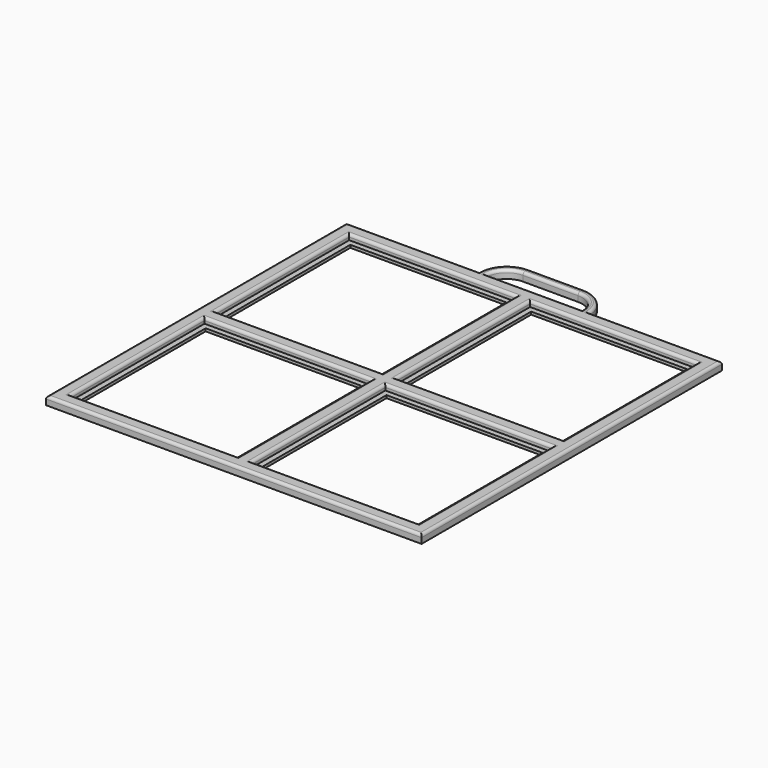
from build123d import *

# Parameters (mm, degrees)
F0_W         = 2.5711264648
F0_H         = 5
F1_DEPTH     = 3
F0_W_2       = 56.75
F0_H_2       = 56.75
F2_DEPTH     = 1
F3_R         = 1
F6_DEPTH     = 3
F7_T1_DEPTH  = 12.5
F7_T3_DEPTH  = 7.5711264648
F7_T5_DEPTH  = 3.5
F7_T8_ANGLE  = 90
F7_T10_ANGLE = 90


# Not quite as in the source:
# - a fillet or chamfer that OpenCascade refuses, or shapes differently, is made with other operations: its cross-section is extruded or revolved along the edge and cut away or added
# - a feature names something its author has since deleted; it is built from what else it names


with BuildPart() as f1:
    # F0 (on Top) → F1 (new body)
    with BuildSketch(Plane.XY):
        Polygon((-63.25, -34.2033516131), (-63.25, 26.5466483869), (-20, 26.5466483869), (-20, 31.5466483869), (-34.125, 31.5466483869), (-68.25, 31.5466483869), (-68.25, -36.7033516131), (0, -36.7033516131), (0, 31.5466483869), (-17.4288735352, 31.5466483869), (-17.4288735352, 26.5466483869), (-2.5, 26.5466483869), (-2.5, -34.2033516131), align=None)
        with Locations((-18.7144367676, 29.0466483869)):
            Rectangle(F0_W, F0_H)
    extrude(amount=F1_DEPTH)

    # F0 (on Top) → F2 (join)
    with BuildSketch(Plane.XY):
        Polygon((-20, 26.5466483869), (-63.25, 26.5466483869), (-63.25, -34.2033516131), (-2.5, -34.2033516131), (-2.5, 26.5466483869), (-17.4288735352, 26.5466483869), align=None)
        with Locations((-32.875, -3.8283516131)):
            Rectangle(F0_W_2, F0_H_2, mode=Mode.SUBTRACT)
    extrude(amount=F2_DEPTH)

    # F3
    f3_edges = [f1.edges().sort_by_distance(p)[0] for p in [
        (-32.875, 26.546648, 3),
        (-63.25, -3.828352, 3),
        (-32.875, -34.203352, 3),
        (-2.5, -3.828352, 3),
        (-34.125, 31.546648, 3),
        (-68.25, -2.578352, 3),
    ]]
    fillet(f3_edges, radius=F3_R)

    # F4: F1 across plane


with BuildPart() as f1_1:
    add(f1.part)
    add(f1.part.mirror(Plane.YZ))

    # F5: F1 across face


with BuildPart() as f1_2:
    add(f1_1.part)
    add(f1_1.part.mirror(Plane(origin=(0, -36.7033516131, 1.4986605371), x_dir=(1, 0, 0), z_dir=(0, -1, 0))))

    # F0 (on Top) → F6 (join)
    with BuildSketch(Plane.XY):
        with BuildLine():
            ThreePointArc((-10, 41.5466483869), (-17.0710678119, 38.6177161988), (-20, 31.5466483869))
            Line((-20, 31.5466483869), (-17.4288735352, 31.5466483869))
            ThreePointArc((-17.4288735352, 31.5466483869), (-15.2530068533, 36.7996552402), (-10, 38.9755219221))
            Line((-10, 38.9755219221), (0, 38.9755219221))
            Line((0, 38.9755219221), (0, 41.5466483869))
            Line((0, 41.5466483869), (-10, 41.5466483869))
        make_face()
        with Locations((-18.7144367676, 29.0466483869)):
            Rectangle(F0_W, F0_H)
    extrude(amount=F6_DEPTH)

    # F7: fillet of radius 1 on 4 edges, made by hand

    # F7_s2 → F7_t1 (cut)
    with BuildSketch(Plane.YZ.offset(-10)):
        with BuildLine():
            ThreePointArc((39.9755219221, 3), (39.2684151409, 2.7071067812), (38.9755219221, 2))
            Line((38.9755219221, 2), (38.9755219221, 3))
            Line((38.9755219221, 3), (39.9755219221, 3))
        make_face()
        with BuildLine():
            ThreePointArc((40.5466483869, 3), (41.2537551681, 2.7071067812), (41.5466483869, 2))
            Line((41.5466483869, 2), (41.5466483869, 3))
            Line((41.5466483869, 3), (40.5466483869, 3))
        make_face()
    extrude(amount=F7_T1_DEPTH, mode=Mode.SUBTRACT)

    # F7_s4 → F7_t3 (cut)
    with BuildSketch(Plane.YZ.offset(-22.5)):
        with BuildLine():
            ThreePointArc((27.5466483869, 3), (26.8395416057, 2.7071067812), (26.5466483869, 2))
            Line((26.5466483869, 2), (26.5466483869, 3))
            Line((26.5466483869, 3), (27.5466483869, 3))
        make_face()
    extrude(amount=F7_T3_DEPTH, mode=Mode.SUBTRACT)

    # F7_s6 → F7_t5 (cut)
    with BuildSketch(Plane.XZ.offset(-31.5466483869)):
        with BuildLine():
            ThreePointArc((-19, 3), (-19.7071067812, 2.7071067812), (-20, 2))
            Line((-20, 2), (-20, 3))
            Line((-20, 3), (-19, 3))
        make_face()
        with BuildLine():
            ThreePointArc((-18.4288735352, 3), (-17.721766754, 2.7071067812), (-17.4288735352, 2))
            Line((-17.4288735352, 2), (-17.4288735352, 3))
            Line((-17.4288735352, 3), (-18.4288735352, 3))
        make_face()
    extrude(amount=F7_T5_DEPTH, mode=Mode.SUBTRACT)

    # F7_s7 → F7_t8 (revolve, cut)
    with BuildSketch(Plane.XZ.offset(-31.5466483869)):
        with BuildLine():
            ThreePointArc((-18.4288735352, 3), (-17.721766754, 2.7071067812), (-17.4288735352, 2))
            Line((-17.4288735352, 2), (-17.4288735352, 3))
            Line((-17.4288735352, 3), (-18.4288735352, 3))
        make_face()
    revolve(axis=Axis((-10, 31.5466483869, 3), (0, 0, -1)), revolution_arc=F7_T8_ANGLE, mode=Mode.SUBTRACT)

    # F7_s9 → F7_t10 (revolve, cut)
    with BuildSketch(Plane.YZ.offset(-10)):
        with BuildLine():
            ThreePointArc((40.5466483869, 3), (41.2537551681, 2.7071067812), (41.5466483869, 2))
            Line((41.5466483869, 2), (41.5466483869, 3))
            Line((41.5466483869, 3), (40.5466483869, 3))
        make_face()
    revolve(axis=Axis((-10, 31.5466483869, 3), (0, 0, 1)), revolution_arc=F7_T10_ANGLE, mode=Mode.SUBTRACT)

    # F8: F1 across plane


with BuildPart() as f1_3:
    add(f1_2.part)
    add(f1_2.part.mirror(Plane.YZ))


solid = f1_3.part
